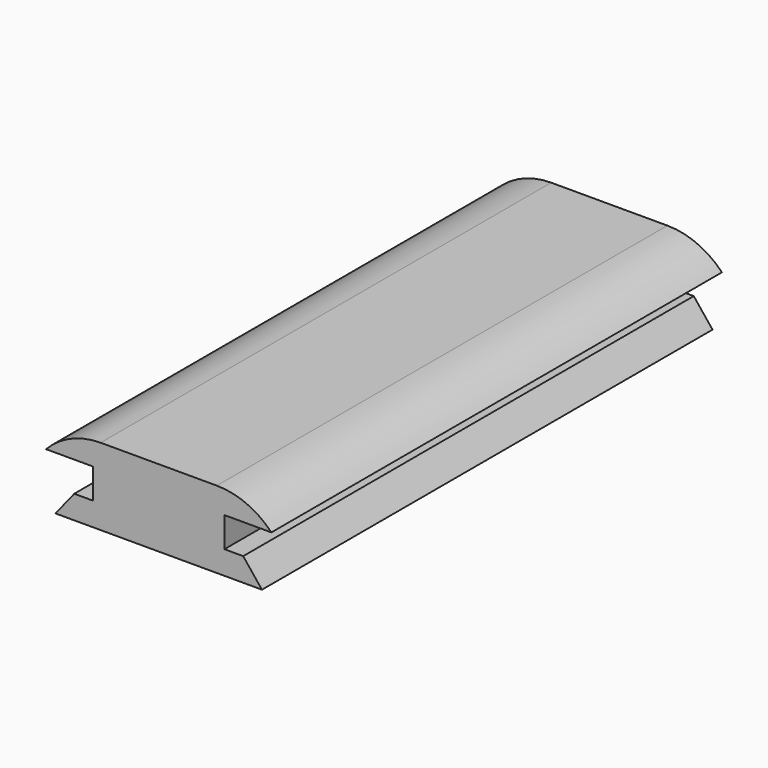
from build123d import *

# Parameters (mm, degrees)
F0_W        = 35
F0_H        = 8
F1_DEPTH    = 150
F2_T1_DEPTH = 197.5947518654


# Not quite as in the source:
# - a fillet or chamfer that OpenCascade refuses, or shapes differently, is made with other operations: its cross-section is extruded or revolved along the edge and cut away or added


with BuildPart() as f1:
    # F0 (on Front) → F1 (new body)
    with BuildSketch(Plane.XZ):
        with Locations((17.5, 4)):
            Rectangle(F0_W, F0_H)
        Polygon((35, 0), (0, 0), (-5, 0), (-10, -6.2449979984), (45, -6.2449979984), (40, 0), align=None)
        Polygon((-12.5, 8), (0, 8), (35, 8), (47.5, 8), (42.5, 14.2449979984), (-7.5, 14.2449979984), align=None)
    extrude(amount=F1_DEPTH)

    # F2: fillet of radius 20 on 2 edges, made by hand

    # F2_s2 → F2_t1 (cut)
    with BuildSketch(Plane.XZ.offset(-23.7973759327)):
        with BuildLine():
            ThreePointArc((2.0189503731, 14.2449979984), (-5.8835796005, 12.6175323912), (-12.5, 8))
            Line((-12.5, 8), (-7.5, 14.2449979984))
            Line((-7.5, 14.2449979984), (2.0189503731, 14.2449979984))
        make_face()
        with BuildLine():
            ThreePointArc((47.5, 8), (40.8835796005, 12.6175323912), (32.9810496269, 14.2449979984))
            Line((32.9810496269, 14.2449979984), (42.5, 14.2449979984))
            Line((42.5, 14.2449979984), (47.5, 8))
        make_face()
    extrude(amount=F2_T1_DEPTH, mode=Mode.SUBTRACT)


solid = f1.part
